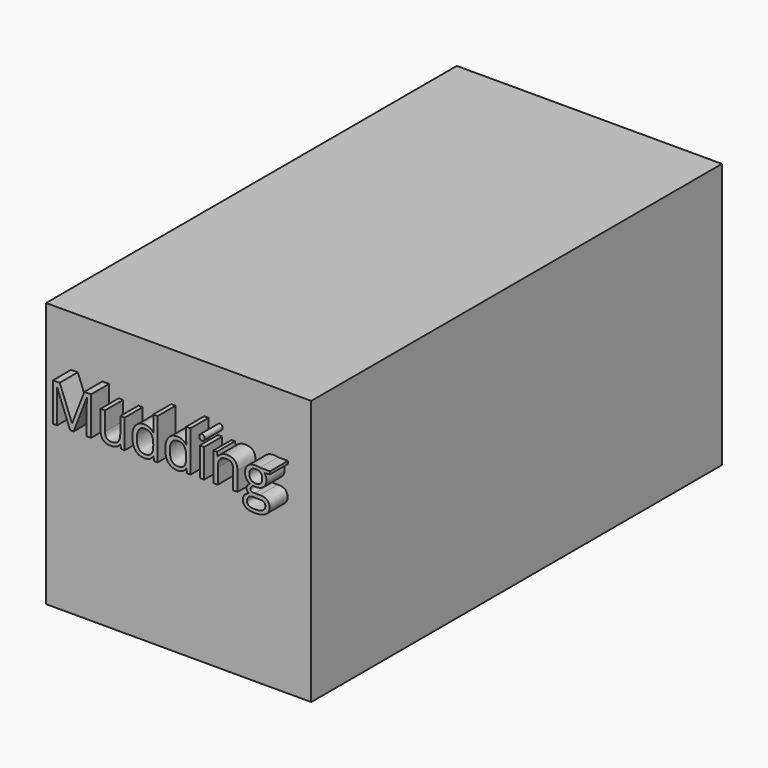
from build123d import *

# Parameters (mm, degrees)
F0_W         = 298.45
F0_H         = 298.45
F1_DEPTH     = 577.85
F2_TEXT_SIZE = 60.5099571934
F3_DEPTH     = 25.4


# Not quite as in the source:
# - Text() gives the source's letters only with a copy of the font that has no kerning and outlines rounded to 1/6400 em; it was checked with that copy


with BuildPart() as f1:
    # F0 (on Front) → F1 (new body)
    with BuildSketch(Plane.XZ):
        Rectangle(F0_W, F0_H)
    extrude(amount=F1_DEPTH)

    # F2 (on face) → F3 (join)
    with BuildSketch(Plane.XZ.offset(577.85)):
        with Locations((-127, 48.9136632376)):
            Text('Mudding', F2_TEXT_SIZE, font='Open Sans', text_align=(TextAlign.LEFT, TextAlign.BOTTOM))
    extrude(amount=F3_DEPTH)


solid = f1.part
